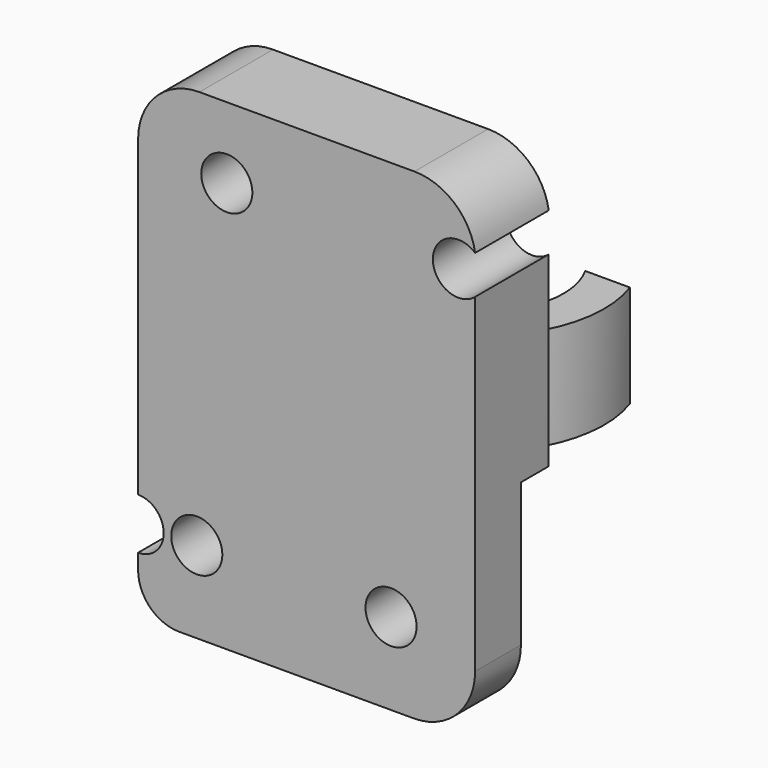
from build123d import *

# Parameters (mm, degrees)
F1_DEPTH     = 20
F3_DEPTH     = 10
F4_R         = 1.25
F5_DEPTH     = 2.2
F7_DEPTH     = 10
F9_R         = 1.25
F10_DEPTH    = 28.001
F11_R        = 2
F14_DEPTH    = 1.5
F16_W        = 20
F16_H        = 10
F17_DEPTH    = 26.7
F19_R        = 1.25
F20_DEPTH    = 32.1
F22_W        = 20
F22_H        = 9.2705127583
F23_DEPTH    = 6.9
F24_DEPTH    = 2.9
F25_R        = 1.25
F26_DEPTH    = 12.5
F27_W        = 15.1660433039
F27_H        = 51.5122525394
F28_DEPTH    = 40.7
F29_W        = 35.2513279067
F29_H        = 19.1500885412
F30_DEPTH    = 12.5
F31_T1_DEPTH = 17.8
F31_T3_DEPTH = 19.5
F31_T5_DEPTH = 19.3219931649


# Not quite as in the source:
# - a fillet or chamfer that OpenCascade refuses, or shapes differently, is made with other operations: its cross-section is extruded or revolved along the edge and cut away or added


with BuildPart() as f1:
    # F0 (on Top) → F1 (new body)
    with BuildSketch(Plane.XY):
        with BuildLine():
            Line((-17.4218026286, 7.8075558554), (-19.6106751933, 7.8075558554))
            ThreePointArc((-19.6106751933, 7.8075558554), (-13.947676921, -0.1749805422), (-8.2846786486, 7.8075558554))
            Line((-8.2846786486, 7.8075558554), (-10.4735512133, 7.8075558554))
            ThreePointArc((-10.4735512133, 7.8075558554), (-13.947676921, 1.8250194578), (-17.4218026286, 7.8075558554))
        make_face()
    extrude(amount=F1_DEPTH)

    # F2 (on Top) → F3 (join, symmetric)
    with BuildSketch(Plane.XY):
        Polygon((-3.947676921, 1.8250194578), (-13.947676921, 1.8250194578), (-23.947676921, 1.8250194578), (-23.947676921, -1.1749805422), (-3.947676921, -1.1749805422), align=None)
    extrude(amount=F3_DEPTH, both=True)

    # F4 (on Front) → F5 (cut, symmetric)
    with BuildSketch(Plane.XZ):
        with Locations((-11.5779312328, -6)):
            Circle(F4_R)
        with Locations((-21.0779312328, -6)):
            Circle(F4_R)
    extrude(amount=F5_DEPTH, both=True, mode=Mode.SUBTRACT)

    # F6 (on face) → F7 (join, through all)
    with BuildSketch(Plane.XY.offset(10)):
        with BuildLine():
            Line((-3.947676921, 1.8250194578), (-9.475540966, 1.8250194578))
            ThreePointArc((-9.475540966, 1.8250194578), (-13.947676921, -0.1749805422), (-18.419812876, 1.8250194578))
            Line((-18.419812876, 1.8250194578), (-23.947676921, 1.8250194578))
            Line((-23.947676921, 1.8250194578), (-23.947676921, -1.1749805422))
            Line((-23.947676921, -1.1749805422), (-3.947676921, -1.1749805422))
            Line((-3.947676921, -1.1749805422), (-3.947676921, 1.8250194578))
        make_face()
    extrude(amount=F7_DEPTH)

    # F9 (on offset) → F10 (cut, through all)
    with BuildSketch(Plane(origin=(0, 26.8250194578, 0), x_dir=(-1, 0, 0), z_dir=(0, 1, 0))):
        with Locations((23.947676921, -6)):
            Circle(F9_R)
        with Locations((3.947676921, -6)):
            Circle(F9_R)
    extrude(amount=-F10_DEPTH, mode=Mode.SUBTRACT)

    # F11
    f11_edges = [f1.edges().sort_by_distance(p)[0] for p in [
        (-23.947677, 0.325019, -10),
        (-3.947677, 0.325019, -10),
    ]]
    fillet(f11_edges, radius=F11_R)

    # F13 (on offset) → F14 (join)
    with BuildSketch(Plane.XZ.offset(1.1749805422)):
        with BuildLine():
            ThreePointArc((-23.947676921, -4.75), (-22.697676921, -6), (-23.947676921, -7.25))
            Line((-23.947676921, -7.25), (-23.947676921, -8))
            ThreePointArc((-23.947676921, -8), (-23.3618904833, -9.4142135624), (-21.947676921, -10))
            Line((-21.947676921, -10), (-5.947676921, -10))
            ThreePointArc((-5.947676921, -10), (-4.5334633586, -9.4142135624), (-3.947676921, -8))
            Line((-3.947676921, -8), (-3.947676921, -7.25))
            ThreePointArc((-3.947676921, -7.25), (-5.197676921, -6), (-3.947676921, -4.75))
            Line((-3.947676921, -4.75), (-3.947676921, 20))
            Line((-3.947676921, 20), (-23.947676921, 20))
            Line((-23.947676921, 20), (-23.947676921, -4.75))
        make_face()
    extrude(amount=F14_DEPTH)

    # F16 (on offset) → F17 (cut)
    with BuildSketch(Plane(origin=(0, 26.8250194578, 0), x_dir=(-1, 0, 0), z_dir=(0, 1, 0))):
        with Locations((13.947676921, -5)):
            Rectangle(F16_W, F16_H)
    extrude(amount=-F17_DEPTH, mode=Mode.SUBTRACT)

    # F19 (on offset) → F20 (cut)
    with BuildSketch(Plane.XZ.offset(25)):
        with Locations((-11.5779312328, -6)):
            Circle(F19_R)
        with Locations((-21.0779312328, -6)):
            Circle(F19_R)
    extrude(amount=-F20_DEPTH, mode=Mode.SUBTRACT)

    # F22 (on offset) → F23 (cut)
    with BuildSketch(Plane.XY.offset(11.9)):
        with Locations((-13.947676921, 6.460275837)):
            Rectangle(F22_W, F22_H)
    extrude(amount=-F23_DEPTH, mode=Mode.SUBTRACT)

    # F22 (on offset) → F24 (cut)
    with BuildSketch(Plane.XY.offset(11.9)):
        with Locations((-13.947676921, 6.460275837)):
            Rectangle(F22_W, F22_H)
    extrude(amount=F24_DEPTH, mode=Mode.SUBTRACT)

    # F25 (on offset) → F26 (cut, symmetric)
    with BuildSketch(Plane(origin=(0, 1.8250194578, 0), x_dir=(-1, 0, 0), z_dir=(0, 1, 0))):
        with Locations((8.2846786486, 10.0688289385)):
            Circle(F25_R)
        with Locations((19.6106751933, 10.0688289385)):
            Circle(F25_R)
    extrude(amount=F26_DEPTH, both=True, mode=Mode.SUBTRACT)

    # F27 (on offset) → F28 (cut)
    with BuildSketch(Plane(origin=(0, 26.8250194578, 0), x_dir=(-1, 0, 0), z_dir=(0, 1, 0))):
        with Locations((-0.11521345, 4.9743577838)):
            Rectangle(F27_W, F27_H)
    extrude(amount=-F28_DEPTH, mode=Mode.SUBTRACT)

    # F29 (on face) → F30 (cut, symmetric)
    with BuildSketch(Plane(origin=(0, 1.8250194578, 0), x_dir=(-1, 0, 0), z_dir=(0, 1, 0))):
        with Locations((16.3581850356, 23.1292308308)):
            Rectangle(F29_W, F29_H)
    extrude(amount=F30_DEPTH, both=True, mode=Mode.SUBTRACT)

    # F31: fillet of radius 3 on 3 edges, made by hand

    # F31_s2 → F31_t1 (cut)
    with BuildSketch(Plane.XZ.offset(-7.6250194578)):
        with BuildLine():
            ThreePointArc((-7.4678082019, -7), (-8.3464878583, -9.1213203436), (-10.4678082019, -10))
            Line((-10.4678082019, -10), (-7.4678082019, -10))
            Line((-7.4678082019, -10), (-7.4678082019, -7))
        make_face()
    extrude(amount=F31_T1_DEPTH, mode=Mode.SUBTRACT)

    # F31_s4 → F31_t3 (cut)
    with BuildSketch(Plane.XZ.offset(-9.3250194578)):
        with BuildLine():
            ThreePointArc((-20.947676921, 13.5541865602), (-23.0689972645, 12.6755069038), (-23.947676921, 10.5541865602))
            Line((-23.947676921, 10.5541865602), (-23.947676921, 13.5541865602))
            Line((-23.947676921, 13.5541865602), (-20.947676921, 13.5541865602))
        make_face()
    extrude(amount=F31_T3_DEPTH, mode=Mode.SUBTRACT)

    # F31_s6 → F31_t5 (cut)
    with BuildSketch(Plane.XZ.offset(-9.2360160403)):
        with BuildLine():
            ThreePointArc((-10.4322068349, 13.5541865602), (-8.4805938304, 12.8326085319), (-7.4678082019, 11.0149910141))
            Line((-7.4678082019, 11.0149910141), (-7.4678082019, 13.5541865602))
            Line((-7.4678082019, 13.5541865602), (-10.4322068349, 13.5541865602))
        make_face()
    extrude(amount=F31_T5_DEPTH, mode=Mode.SUBTRACT)


solid = f1.part
